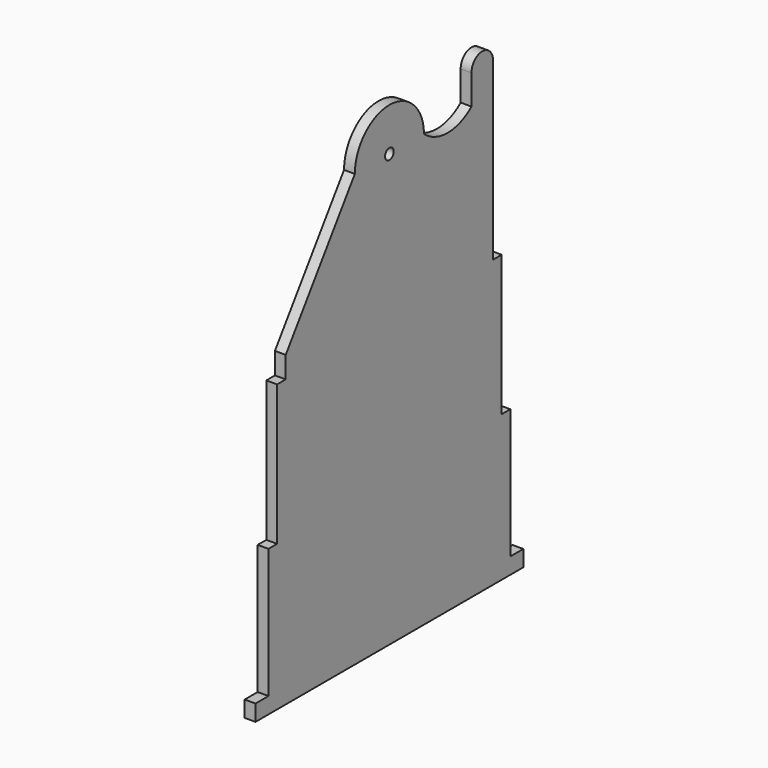
from build123d import *

# Parameters (mm, degrees)
F0_R     = 3.175
F1_DEPTH = 6.35


# Not quite as in the source:
# - ends of sketch curves that miss each other by under 0.0002 mm in the source are joined


with BuildPart() as f1:
    # F0 (on Right) → F1 (new body)
    with BuildSketch(Plane.YZ):
        with BuildLine():
            Line((-88.9, -53.975), (-88.9, -130.175))
            Line((-88.9, -130.175), (-98.425, -130.175))
            Line((-98.425, -130.175), (-98.425, -139.7))
            Line((-98.425, -139.7), (98.425, -139.7))
            Line((98.425, -139.7), (98.425, -130.175))
            Line((98.425, -130.175), (88.9, -130.175))
            Line((88.9, -130.175), (88.9, -53.975))
            Line((88.9, -53.975), (82.55, -53.975))
            Line((82.55, -53.975), (82.55, 28.575))
            Line((82.55, 28.575), (76.2, 28.575))
            Line((76.2, 28.575), (76.2, 34.925))
            Line((76.2, 34.925), (76.2, 131.7625))
            ThreePointArc((76.2, 131.7625), (68.2625, 139.7), (60.325, 131.7625))
            Line((60.325, 131.7625), (60.325, 114.3))
            ThreePointArc((60.325, 114.3), (42.8625, 107.8115954), (25.3999938624, 114.299992881))
            ThreePointArc((25.3999938624, 114.299992881), (0, 139.7), (-25.4, 114.3))
            Line((-25.4, 114.3), (-76.2, 41.275))
            Line((-76.2, 41.275), (-76.2, 28.575))
            Line((-76.2, 28.575), (-82.55, 28.575))
            Line((-82.55, 28.575), (-82.55, -53.975))
            Line((-82.55, -53.975), (-88.9, -53.975))
        make_face()
        with Locations((0, 114.3)):
            Circle(F0_R, mode=Mode.SUBTRACT)
    extrude(amount=F1_DEPTH)


solid = f1.part
